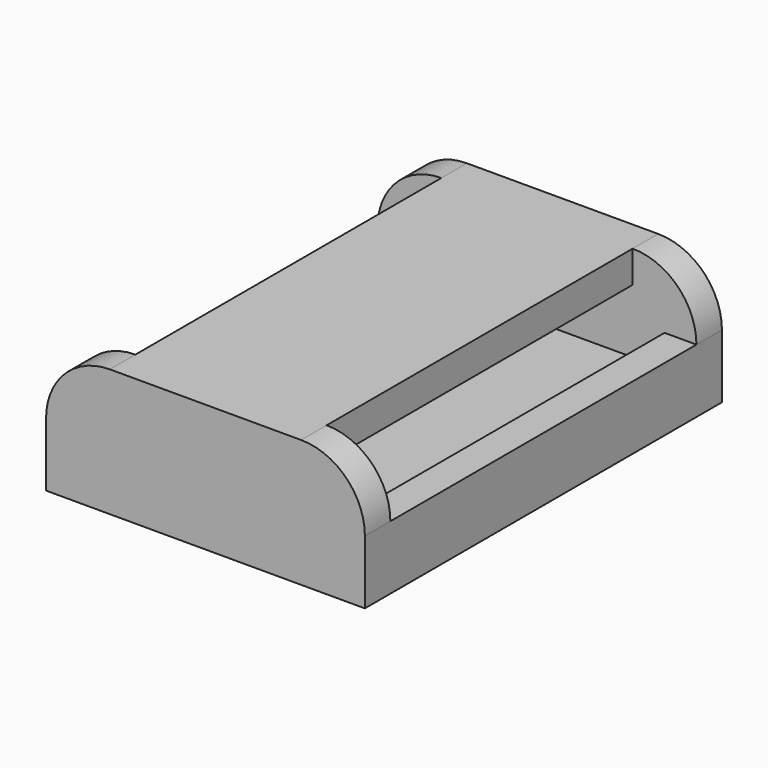
from build123d import *

# Parameters (mm, degrees)
F0_W     = 25
F0_H     = 35
F1_DEPTH = 5
F2_W     = 25
F2_H     = 35
F3_DEPTH = 10
F4_R     = 5
F5_T     = 2.5


# Not quite as in the source:
# - a shell that OpenCascade refuses in one call is made with other operations: the cavity is built on its own and cut out


with BuildPart() as f1:
    # F0 (on Top) → F1 (new body)
    with BuildSketch(Plane.XY):
        Rectangle(F0_W, F0_H)
    extrude(amount=F1_DEPTH)

    # F2 (on Top) → F3 (join)
    with BuildSketch(Plane.XY):
        Rectangle(F2_W, F2_H)
    extrude(amount=F3_DEPTH)

    # F4
    f4_edges = [f1.edges().sort_by_distance(p)[0] for p in [
        (-12.5, 0, 10),
        (12.5, 0, 10),
    ]]
    fillet(f4_edges, radius=F4_R)

    # F5: shell of thickness 2.5, made by hand


with BuildPart() as f5_core1:
    # F5_t2: copy of F1
    add(f1.part)

    # the walls: a layer under each face that stays
    f5_faces = [f5_core1.faces().sort_by_distance(p)[0] for p in [
        (0, -17.5, 5),
        (-12.5, 0, 2.5),
        (0, 0, 0),
        (0, 0, 10),
        (12.5, 0, 2.5),
        (0, 17.5, 5),
    ]]
    thicken(f5_faces, amount=-F5_T, mode=Mode.SUBTRACT)


with BuildPart() as f1_1:
    add(f1.part)

    # what is left inside the walls is the cavity
    f5_cavity = [f5_core1.part.solids().sort_by_distance(p)[0] for p in [
        (0, -5, 2.525),
    ]]
    add(f5_cavity, mode=Mode.SUBTRACT)


solid = f1_1.part
